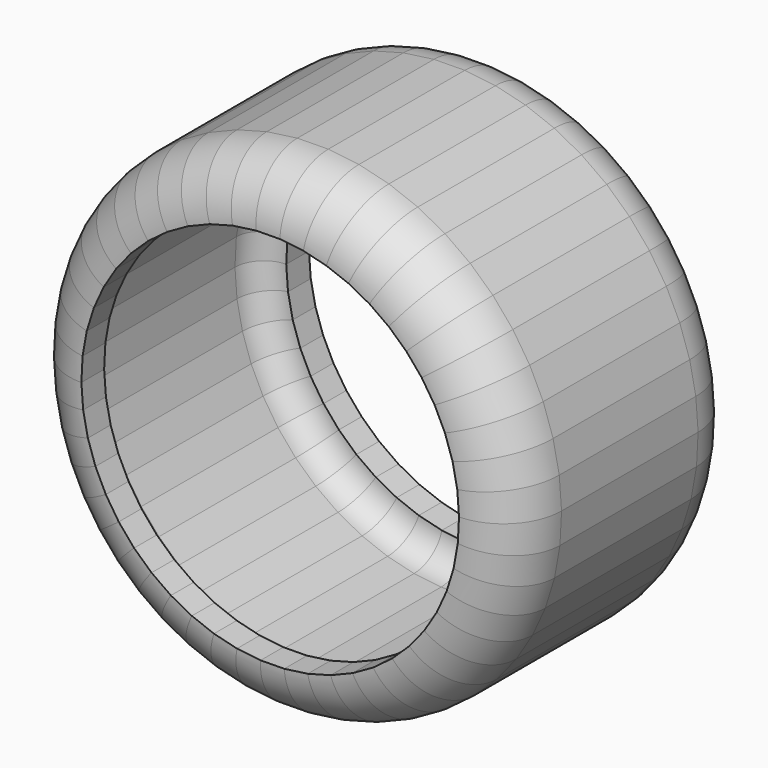
from build123d import *

# Parameters (mm, degrees)
F1_DEPTH = 25.4
F2_R     = 5.08
F3_T     = -2.54


# Not quite as in the source:
# - a shell that OpenCascade refuses in one call is made with other operations: the cavity is built on its own and cut out


with BuildPart() as f1:
    # F0 (on Front) → F1 (new body)
    with BuildSketch(Plane.XZ):
        Polygon((-51.8681113449, 34.9863301754), (-49.6573708951, 36.6324856877), (-47.6703807875, 38.5427400213), (-45.9384770428, 40.6869673242), (-44.4889728179, 43.0313518509), (-43.3447276601, 45.5389212569), (-42.5237869993, 48.1701296748), (-42.0390975599, 50.883481376), (-41.8983031841, 53.6361851833), (-42.1036242832, 56.3848293133), (-42.6518228208, 59.0860660061), (-43.5342533785, 61.6972951454), (-44.7369994993, 64.1773360878), (-46.2410931584, 66.4870771061), (-48.0228139003, 68.5900922047), (-50.0540629245, 70.4532155793), (-52.3028062205, 72.0470646611), (-54.7335797632, 73.3465034982), (-57.3080488017, 74.3310391637), (-59.9856124214, 74.9851449422), (-62.7240438446, 75.2985051947), (-65.4801563717, 75.2661780428), (-68.2104844619, 74.8886733051), (-70.8719692101, 74.1719444567), (-73.422637412, 73.1272947399), (-75.8222635063, 71.7711989045), (-78.0330039561, 70.1250433922), (-80.0199940638, 68.2147890586), (-81.7518978084, 66.0705617557), (-83.2014020333, 63.726177229), (-84.3456471911, 61.218607823), (-85.1665878519, 58.5873994051), (-85.6512772913, 55.8740477039), (-85.7920716671, 53.1213438966), (-85.5867505681, 50.3726997666), (-85.0385520304, 47.6714630738), (-84.1561214727, 45.0602339345), (-82.9533753519, 42.5801929922), (-81.4492816928, 40.2704519738), (-79.6675609509, 38.1674368752), (-77.6363119267, 36.3043135007), (-75.3875686307, 34.7104644188), (-72.956795088, 33.4110255817), (-70.3823260495, 32.4264899162), (-67.7047624298, 31.7723841377), (-64.9663310067, 31.4590238853), (-62.2102184795, 31.4913510371), (-59.4798903893, 31.8688557748), (-56.8184056411, 32.5855846232), (-54.2677374392, 33.6302343401), align=None)
    extrude(amount=F1_DEPTH)

    # F2
    f2_edges = [f1.edges().sort_by_distance(p)[0] for p in [
        (-85.312651, -25.4, 49.022081),
        (-84.597337, -25.4, 46.365849),
        (-83.554748, -25.4, 43.820213),
        (-82.201329, -25.4, 41.425322),
        (-80.558421, -25.4, 39.218944),
        (-78.651936, -25.4, 37.235875),
        (-76.51194, -25.4, 35.507389),
        (-74.172182, -25.4, 34.060745),
        (-71.669561, -25.4, 32.918758),
        (-69.043544, -25.4, 32.099437),
        (-66.335547, -25.4, 31.615704),
        (-63.588275, -25.4, 31.475187),
        (-60.845054, -25.4, 31.680103),
        (-58.149148, -25.4, 32.22722),
        (-55.543072, -25.4, 33.107909),
        (-53.067924, -25.4, 34.308282),
        (-50.762741, -25.4, 35.809408),
        (-48.663876, -25.4, 37.587613),
        (-46.804429, -25.4, 39.614854),
        (-45.213725, -25.4, 41.85916),
        (-43.91685, -25.4, 44.285137),
        (-42.934257, -25.4, 46.854525),
        (-42.281442, -25.4, 49.526806),
        (-41.9687, -25.4, 52.259833),
        (-42.000964, -25.4, 55.010507),
        (-42.377724, -25.4, 57.735448),
        (-43.093038, -25.4, 60.391681),
        (-44.135626, -25.4, 62.937316),
        (-45.489046, -25.4, 65.332207),
        (-47.131954, -25.4, 67.538585),
        (-49.038438, -25.4, 69.521654),
        (-51.178435, -25.4, 71.25014),
        (-53.518193, -25.4, 72.696784),
        (-56.020814, -25.4, 73.838771),
        (-58.646831, -25.4, 74.658092),
        (-61.354828, -25.4, 75.141825),
        (-64.1021, -25.4, 75.282342),
        (-66.84532, -25.4, 75.077426),
        (-69.541227, -25.4, 74.530309),
        (-72.147303, -25.4, 73.64962),
        (-74.62245, -25.4, 72.449247),
        (-76.927634, -25.4, 70.948121),
        (-79.026499, -25.4, 69.169916),
        (-80.885946, -25.4, 67.142675),
        (-82.47665, -25.4, 64.898369),
        (-83.773525, -25.4, 62.472393),
        (-84.756118, -25.4, 59.903004),
        (-85.408933, -25.4, 57.230724),
        (-85.721674, -25.4, 54.497696),
        (-85.689411, -25.4, 51.747022),
        (-85.312651, 0, 49.022081),
        (-84.597337, 0, 46.365849),
        (-83.554748, 0, 43.820213),
        (-82.201329, 0, 41.425322),
        (-80.558421, 0, 39.218944),
        (-78.651936, 0, 37.235875),
        (-76.51194, 0, 35.507389),
        (-74.172182, 0, 34.060745),
        (-71.669561, 0, 32.918758),
        (-69.043544, 0, 32.099437),
        (-66.335547, 0, 31.615704),
        (-63.588275, 0, 31.475187),
        (-60.845054, 0, 31.680103),
        (-58.149148, 0, 32.22722),
        (-55.543072, 0, 33.107909),
        (-53.067924, 0, 34.308282),
        (-50.762741, 0, 35.809408),
        (-48.663876, 0, 37.587613),
        (-46.804429, 0, 39.614854),
        (-45.213725, 0, 41.85916),
        (-43.91685, 0, 44.285137),
        (-42.934257, 0, 46.854525),
        (-42.281442, 0, 49.526806),
        (-41.9687, 0, 52.259833),
        (-42.000964, 0, 55.010507),
        (-42.377724, 0, 57.735448),
        (-43.093038, 0, 60.391681),
        (-44.135626, 0, 62.937316),
        (-45.489046, 0, 65.332207),
        (-47.131954, 0, 67.538585),
        (-49.038438, 0, 69.521654),
        (-51.178435, 0, 71.25014),
        (-53.518193, 0, 72.696784),
        (-56.020814, 0, 73.838771),
        (-58.646831, 0, 74.658092),
        (-61.354828, 0, 75.141825),
        (-64.1021, 0, 75.282342),
        (-66.84532, 0, 75.077426),
        (-69.541227, 0, 74.530309),
        (-72.147303, 0, 73.64962),
        (-74.62245, 0, 72.449247),
        (-76.927634, 0, 70.948121),
        (-79.026499, 0, 69.169916),
        (-80.885946, 0, 67.142675),
        (-82.47665, 0, 64.898369),
        (-83.773525, 0, 62.472393),
        (-84.756118, 0, 59.903004),
        (-85.408933, 0, 57.230724),
        (-85.721674, 0, 54.497696),
        (-85.689411, 0, 51.747022),
    ]]
    fillet(f2_edges, radius=F2_R)

    # F3: a shell. OpenCascade refuses it in one call, so the cavity is built on its own and cut out:
    # the body offset inwards by the wall thickness, plus a prism from it out through each open face.
    f3_core = offset(f1.part, amount=F3_T, mode=Mode.PRIVATE)
    f3_exits = [f3_core.faces().sort_by_distance(p)[0] for p in [
        (-63.845187, -22.86, 53.378765),
        (-63.845187, -2.54, 53.378765),
    ]]
    add(f3_core, mode=Mode.SUBTRACT)
    extrude(f3_exits, amount=-F3_T, mode=Mode.SUBTRACT)


solid = f1.part
